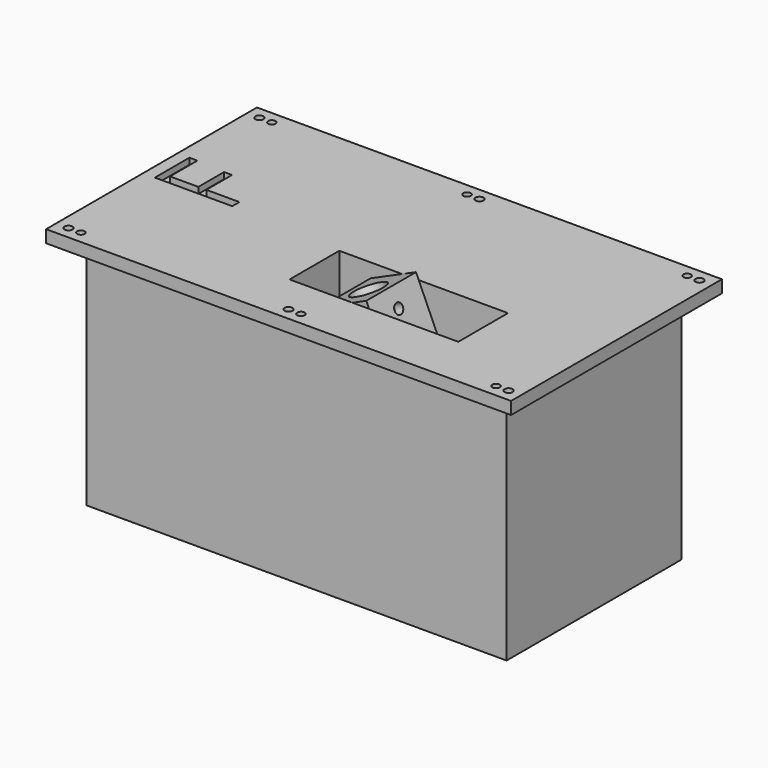
from build123d import *

# Parameters (mm, degrees)
F0_W         = 374
F0_H         = 212
F1_DEPTH     = 10
F2_W         = 15
F2_H         = 65
F3_DEPTH     = 187
F4_W         = 135.7326568991
F4_H         = 50
F5_DEPTH     = 50
F7_D         = 6
F7_DEPTH     = 10
F7_TIP       = 1.8025818571
F8_D         = 6.5
F8_DEPTH     = 10
F8_TIP       = 1.9527970118
F9_TEXT_SIZE = 87.1982658282
F10_DEPTH    = 5
F13_DEPTH    = 25
F14_R        = 13
F15_DEPTH    = 33
F16_R        = 4.1
F17_DEPTH    = 47


# Not quite as in the source:
# - Text() gives the source's letters only with a copy of the font that has no kerning and outlines rounded to 1/6400 em; it was checked with that copy


with BuildPart() as f1:
    # F0 (on Top) → F1 (new body)
    with BuildSketch(Plane.XY):
        Rectangle(F0_W, F0_H)
    extrude(amount=F1_DEPTH)

    # F2 (on face) → F3 (join)
    with BuildSketch(Plane(origin=(0, 0, 0), x_dir=(1, 0, 0), z_dir=(0, 0, -1))):
        Polygon((-169, -88), (169, -88), (169, 88), (-169, 88), (-169, 3.7), (-169, -61.3), align=None)
        with Locations((-176.5, -28.8)):
            Rectangle(F2_W, F2_H)
    extrude(amount=F3_DEPTH)

    # F4 (on face) → F5 (cut)
    with BuildSketch(Plane.XY.offset(10)):
        with Locations((43, -38.9)):
            Rectangle(F4_W, F4_H)
    extrude(amount=-F5_DEPTH, mode=Mode.SUBTRACT)

    # F7
    with Locations(Plane.XY.offset(10)):
        with Locations((-167, 96), (-167, -96), (167, -96), (167, 96), (-10, 96), (10, -96)):
            Hole(F7_D / 2, depth=F7_DEPTH)
            with Locations((0, 0, -(F7_DEPTH + F7_TIP / 2))):  # 118° drill point
                Cone(0, F7_D / 2, F7_TIP, mode=Mode.SUBTRACT)

    # F8
    with Locations(Plane.XY.offset(10)):
        with Locations((-177, 96), (-177, -96), (0, -96), (0, 96), (177, 96), (177, -96)):
            Hole(F8_D / 2, depth=F8_DEPTH)
            with Locations((0, 0, -(F8_DEPTH + F8_TIP / 2))):  # 118° drill point
                Cone(0, F8_D / 2, F8_TIP, mode=Mode.SUBTRACT)

    # F9 (on face) → F10 (cut)
    with BuildSketch(Plane.XY.offset(10)):
        with Locations(Location((-115.21140486, -17.1157363802), (0, 0, 90))):
            Text('F', F9_TEXT_SIZE, font='Open Sans', text_align=(TextAlign.LEFT, TextAlign.BOTTOM))
    extrude(amount=-F10_DEPTH, mode=Mode.SUBTRACT)

    # F12 (on offset) → F13 (join, symmetric)
    with BuildSketch(Plane.XZ.offset(38.9)):
        Polygon((61.2709091529, -39.8652671385), (36.8667105683, 14.9474603201), (0.3248922626, -1.322005403), (24.7290908471, -56.1347328615), align=None)
    extrude(amount=F13_DEPTH, both=True)

    # F14 (on face) → F15 (cut)
    with BuildSketch(Plane(origin=(0.5449691902, 0, -1.2240208418), x_dir=(0.9135454576, 0, 0.4067366431), z_dir=(-0.4067366431, 0, 0.9135454576))):
        with Locations((19.759095811, -38.9)):
            Circle(F14_R)
    extrude(amount=-F15_DEPTH, mode=Mode.SUBTRACT)

    # F16 (on face) → F17 (cut)
    with BuildSketch(Plane(origin=(36.3217413781, 0, 16.1714811619), x_dir=(0, 1, 0), z_dir=(0.9135454576, 0, 0.4067366431))):
        with Locations((-38.9, -16.3398576191)):
            Circle(F16_R)
    extrude(amount=-F17_DEPTH, mode=Mode.SUBTRACT)


solid = f1.part
